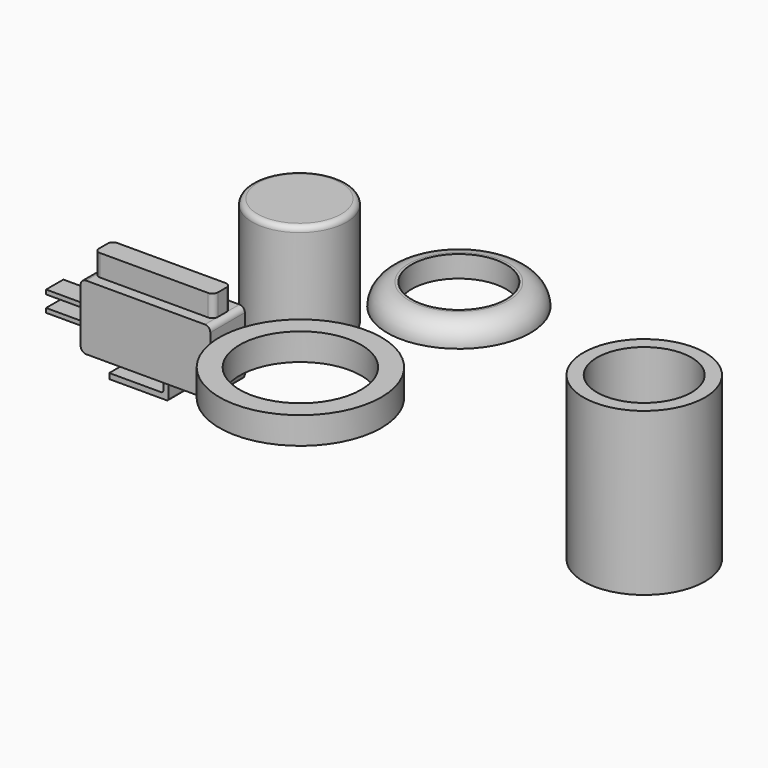
from build123d import *

# Parameters (mm, degrees)
F0_W      = 30.48
F0_H      = 10.16
F1_DEPTH  = 15.24
F2_W      = 5.08
F2_H      = 1.016
F3_DEPTH  = 10.16
F4_W      = 1.27
F4_H      = 5.08
F5_DEPTH  = 5.08
F6_W      = 5.08
F6_H      = 1.27
F7_DEPTH  = 12.7
F8_R      = 0.508
F9_R      = 1.27
F10_W     = 27.94
F10_H     = 5.08
F11_DEPTH = 5.08
F12_R     = 1.27
F13_R     = 14.2875
F13_R_2   = 11.1125
F14_DEPTH = 38.1
F13_R_3   = 16.8275
F15_DEPTH = 5.08
F16_DEPTH = 10.16
F17_DEPTH = 15.24
F18_R     = 1.27
F19_R     = 5.07999
F13_R_4   = 19.05
F20_DEPTH = 6.35


# Not quite as in the source:
# - a fillet or chamfer is up to 0.001 mm smaller than in the source, because OpenCascade refuses the exact size


with BuildPart() as f1:
    # F0 (on Top) → F1 (new body)
    with BuildSketch(Plane.XY):
        with Locations((-45.9272513187, 16.9497304279)):
            Rectangle(F0_W, F0_H)
    extrude(amount=-F1_DEPTH)

    # F2 (on face) → F3 (join)
    with BuildSketch(Plane(origin=(-61.1672513187, 0, 0), x_dir=(0, -1, 0), z_dir=(-1, 0, 0))):
        with Locations((-16.9497304279, -7.112)):
            Rectangle(F2_W, F2_H)
        with Locations((-16.9497304279, -10.922)):
            Rectangle(F2_W, F2_H)
    extrude(amount=F3_DEPTH)

    # F4 (on face) → F5 (join)
    with BuildSketch(Plane(origin=(0, 0, -15.24), x_dir=(1, 0, 0), z_dir=(0, 0, -1))):
        with Locations((-43.1381706691, -16.9497304279)):
            Rectangle(F4_W, F4_H)
    extrude(amount=F5_DEPTH)

    # F6 (on face) → F7 (join)
    with BuildSketch(Plane(origin=(-43.7731706691, 0, 0), x_dir=(0, -1, 0), z_dir=(-1, 0, 0))):
        with Locations((-16.9497304279, -19.685)):
            Rectangle(F6_W, F6_H)
    extrude(amount=F7_DEPTH)

    # F8
    f8_edges = [f1.edges().sort_by_distance(p)[0] for p in [
        (-42.503171, 16.94973, -20.32),
        (-43.773171, 16.94973, -19.05),
    ]]
    fillet(f8_edges, radius=F8_R)

    # F9
    f9_edges = [f1.edges().sort_by_distance(p)[0] for p in [
        (-30.687251, 16.94973, -15.24),
        (-61.167251, 16.94973, -15.24),
        (-30.687251, 16.94973, 0),
        (-61.167251, 16.94973, 0),
    ]]
    fillet(f9_edges, radius=F9_R)

    # F10 (on face) → F11 (join)
    with BuildSketch(Plane.XY):
        with Locations((-45.9272513187, 16.9497304279)):
            Rectangle(F10_W, F10_H)
    extrude(amount=F11_DEPTH)

    # F12
    f12_edges = [f1.edges().sort_by_distance(p)[0] for p in [
        (-31.957251, 14.40973, 2.54),
        (-59.897251, 14.40973, 2.54),
        (-59.897251, 19.48973, 2.54),
        (-31.957251, 19.48973, 2.54),
    ]]
    fillet(f12_edges, radius=F12_R)


with BuildPart() as f14:
    # F13 (on Top) → F14 (new body)
    with BuildSketch(Plane.XY):
        with Locations((43.5843914747, 46.5672239661)):
            Circle(F13_R)
        with Locations((43.5843914747, 46.5672239661)):
            Circle(F13_R_2, mode=Mode.SUBTRACT)
    extrude(amount=-F14_DEPTH)


with BuildPart() as f15:
    # F13 (on Top) → F15 (new body)
    with BuildSketch(Plane.XY):
        with Locations((0, 46.5672239661)):
            Circle(F13_R_3)
        with Locations((0, 46.5672239661)):
            Circle(F13_R_2, mode=Mode.SUBTRACT)
    extrude(amount=F15_DEPTH)

    # F19 (radius 5.08 in the source; OpenCascade refuses exactly that, so slightly less here)
    f19_edges = [f15.edges().sort_by_distance(p)[0] for p in [
        (-16.8275, 46.567224, 5.08),
    ]]
    fillet(f19_edges, radius=F19_R)


with BuildPart() as f16:
    # F13 (on Top) → F16 (new body)
    with BuildSketch(Plane.XY):
        with Locations((-37.4783687294, 46.5672239661)):
            Circle(F13_R_2)
    extrude(amount=F16_DEPTH)

    # F17 (add): a face of the model
    f17_faces = [f16.faces().sort_by_distance(p)[0] for p in [
        (-37.4783687294, 46.5672239661, 0),
    ]]
    extrude(f17_faces, amount=F17_DEPTH)

    # F18
    f18_edges = [f16.edges().sort_by_distance(p)[0] for p in [
        (-48.590869, 46.567224, 10.16),
    ]]
    fillet(f18_edges, radius=F18_R)


with BuildPart() as f20:
    # F13 (on Top) → F20 (new body)
    with BuildSketch(Plane.XY):
        Circle(F13_R_4)
        Circle(F13_R, mode=Mode.SUBTRACT)
    extrude(amount=F20_DEPTH)


solid = Compound([f1.part, f14.part, f15.part, f16.part, f20.part])
